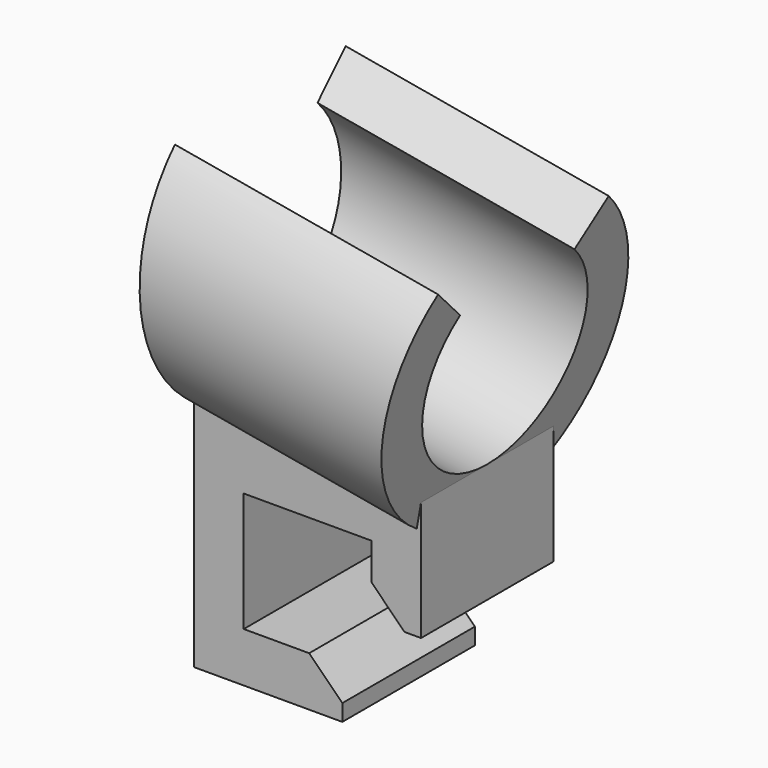
from build123d import *

# Parameters (mm, degrees)
F3_DEPTH  = 14
F5_DEPTH  = 5
F6_SIZE   = 2
F7_DEPTH  = 25
F9_DEPTH  = 51.6
F10_DEPTH = 1.1


# Not quite as in the source:
# - a feature names something its author has since deleted; it is built from what else it names


with BuildPart() as f3:
    # F2 (on line) → F3 (new body)
    with BuildSketch(Plane(origin=(0, 0, 0), x_dir=(0, 1, 0), z_dir=(0.984807753, 0, -0.1736481777))):
        with BuildLine():
            ThreePointArc((4.3133513652, 4.3133513652), (5.6356651483, 2.3343689374), (6.1, 0))
            ThreePointArc((6.1, 0), (-2.3343689374, -5.6356651483), (-4.3133513652, 4.3133513652))
            Line((-4.3133513652, 4.3133513652), (-6.4346717088, 6.4346717088))
            ThreePointArc((-6.4346717088, 6.4346717088), (-3.4824192345, -8.4073037459), (9.1, 0))
            ThreePointArc((9.1, 0), (8.4073037459, 3.4824192345), (6.4346717088, 6.4346717088))
            Line((6.4346717088, 6.4346717088), (4.3133513652, 4.3133513652))
        make_face()
    extrude(amount=F3_DEPTH)

    # F4 (on Front) → F5 (join, symmetric)
    with BuildSketch(Plane.XZ):
        Polygon((-0.9719453416, -8.4384017807), (-0.9719453416, -21.6384017807), (7.9780546584, -21.6384017807), (7.9780546584, -18.6384017807), (2.0280546584, -18.6384017807), (2.0280546584, -11.4384017807), (9.7280546584, -11.4384017807), (9.7280546584, -15.6384017807), (12.7280546584, -15.6384017807), (12.7280546584, -11.4438512443), (12.7280546584, -8.4384017807), align=None)
    extrude(amount=F5_DEPTH, both=True)

    # F6
    f6_edges = [f3.edges().sort_by_distance(p)[0] for p in [
        (9.728055, 0, -15.638402),
        (7.978055, 0, -18.638402),
    ]]
    chamfer(f6_edges, length=F6_SIZE)

    # F7 (add): a face of the model
    f7_faces = [f3.faces().sort_by_distance(p)[0] for p in [
        (-1.1008050308, 0, -6.2429755581),
    ]]
    extrude(f7_faces, amount=F7_DEPTH)

    # F8 (on face) → F9 (cut)
    with BuildSketch(Plane(origin=(-0.9719453416, 0, 0), x_dir=(0, -1, 0), z_dir=(-1, 0, 0))):
        with BuildLine():
            Line((22.6868242025, -11.5467039868), (22.6868242025, 11.5467039868))
            Line((22.6868242025, 11.5467039868), (-22.6868242025, 11.5467039868))
            Line((-22.6868242025, 11.5467039868), (-22.6868242025, -11.5467039868))
            Line((-22.6868242025, -11.5467039868), (-5, -11.5467039868))
            Line((-5, -11.5467039868), (-5, -8.4384017807))
            Line((-5, -8.4384017807), (-3.3040728779, -8.4384017807))
            add(Edge.make_bspline(
                [(-3.3040728779, -8.4384017807), (0, -9.7457887872), (3.3040728779, -8.4384017807)],
                knots=[2.7700160081, 2.7700160081, 2.7700160081, 3.5131692991, 3.5131692991, 3.5131692991], degree=2, weights=[1, 0.9317560477, 1]))
            Line((3.3040728779, -8.4384017807), (5, -8.4384017807))
            Line((5, -8.4384017807), (5, -11.5467039868))
            Line((5, -11.5467039868), (22.6868242025, -11.5467039868))
        make_face()
    extrude(amount=F9_DEPTH, mode=Mode.SUBTRACT)

    # F10 (add): faces of the model
    f10_faces = [f3.faces().sort_by_distance(p)[0] for p in [
        (0.6395749646, -4.4604313904, -8.4384017807),
        (0.6395749646, 4.4604313904, -8.4384017807),
    ]]
    extrude(f10_faces, amount=F10_DEPTH)


solid = f3.part
